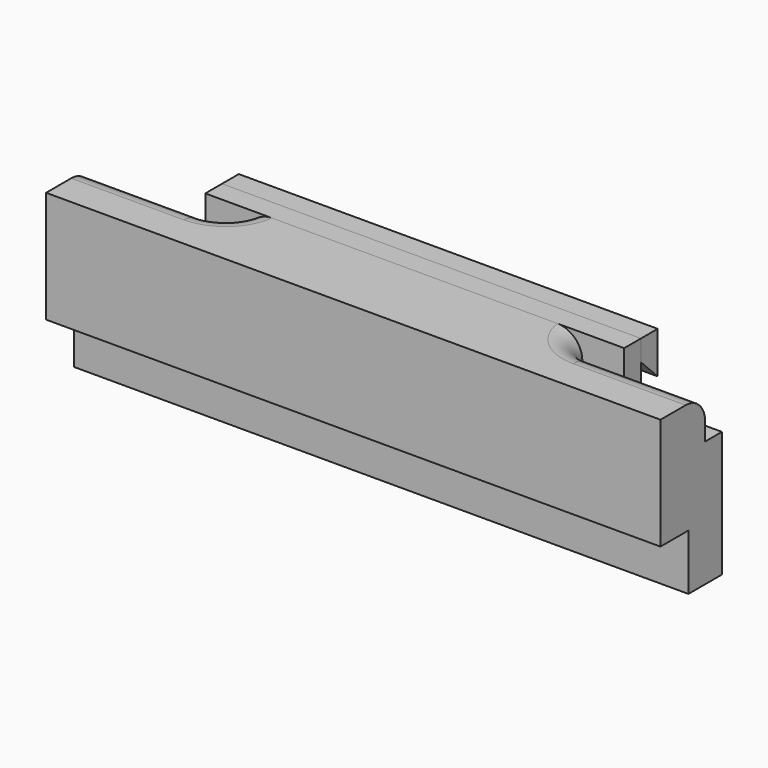
from build123d import *

# Parameters (mm, degrees)
F0_W        = 558.8
F0_H        = 152.4
F1_DEPTH    = 69.85
F2_W        = 558.8
F2_H        = 50.8
F3_DEPTH    = 31.75
F4_W        = 127
F4_H        = 19.05
F5_DEPTH    = 38.1
F6_T1_DEPTH = 99.583610621
F7_R        = 22.225
F9_D        = 5.1054
F9_DEPTH    = 12.7
F9_TIP      = 1.5338169022
F10_W       = 381
F10_H       = 139.7
F11_DEPTH   = 19.05
F13_DEPTH   = 381


# Not quite as in the source:
# - a fillet or chamfer that OpenCascade refuses, or shapes differently, is made with other operations: its cross-section is extruded or revolved along the edge and cut away or added


with BuildPart() as f1:
    # F0 (on Front) → F1 (new body)
    with BuildSketch(Plane.XZ):
        with Locations((279.4, 76.2)):
            Rectangle(F0_W, F0_H)
    extrude(amount=F1_DEPTH)

    # F2 (on face) → F3 (cut)
    with BuildSketch(Plane.XZ.offset(69.85)):
        with Locations((279.4, 25.4)):
            Rectangle(F2_W, F2_H)
    extrude(amount=-F3_DEPTH, mode=Mode.SUBTRACT)

    # F4 (on face) → F5 (cut)
    with BuildSketch(Plane.XY.offset(152.4)):
        with Locations((63.5, -9.525)):
            Rectangle(F4_W, F4_H)
        with Locations((495.3, -9.525)):
            Rectangle(F4_W, F4_H)
    extrude(amount=-F5_DEPTH, mode=Mode.SUBTRACT)

    # F6: fillet of radius 25.4 on 2 edges, made by hand

    # F6_s2 → F6_t1 (join)
    with BuildSketch(Plane.XY.offset(52.816389379)):
        with BuildLine():
            ThreePointArc((102.4065557516, -19.05), (117.9608156183, -13.7304631421), (127, 0))
            Line((127, 0), (127, -19.05))
            Line((127, -19.05), (102.4065557516, -19.05))
        make_face()
        with BuildLine():
            ThreePointArc((431.8, 0), (440.8391843817, -13.7304631421), (456.3934442484, -19.05))
            Line((456.3934442484, -19.05), (431.8, -19.05))
            Line((431.8, -19.05), (431.8, 0))
        make_face()
    extrude(amount=F6_T1_DEPTH)

    # F7
    f7_edges = [f1.edges().sort_by_distance(p)[0] for p in [
        (51.203278, -19.05, 152.4),
        (440.839184, -13.730463, 152.4),
        (507.596722, -19.05, 152.4),
        (117.960816, -13.730463, 152.4),
    ]]
    fillet(f7_edges, radius=F7_R)

    # F9
    with Locations(Plane(origin=(0, 0, 0), x_dir=(-1, 0, 0), z_dir=(0, 1, 0))):
        with Locations((-439.7375, 49.2125), (-437.35625, 98.425), (-332.58125, 49.2125), (-278.60625, 108.74375), (-225.425, 49.2125), (-119.0625, 49.2125), (-114.3, 98.425)):
            Hole(F9_D / 2, depth=F9_DEPTH)
            with Locations((0, 0, -(F9_DEPTH + F9_TIP / 2))):  # 118° drill point
                Cone(0, F9_D / 2, F9_TIP, mode=Mode.SUBTRACT)


with BuildPart() as f11:
    # F10 (on face) → F11 (new body)
    with BuildSketch(Plane(origin=(0, 0, 0), x_dir=(-1, 0, 0), z_dir=(0, 1, 0))):
        with Locations((-279.4, 82.55)):
            Rectangle(F10_W, F10_H)
    extrude(amount=F11_DEPTH)


with BuildPart() as f13:
    # F12 (on face) → F13 (new body)
    with BuildSketch(Plane.YZ.offset(469.9)):
        Polygon((38.1, 152.4), (19.05, 152.4), (19.05, 133.35), (38.1, 114.3), align=None)
    extrude(amount=-F13_DEPTH)


solid = Compound([f1.part, f11.part, f13.part])
